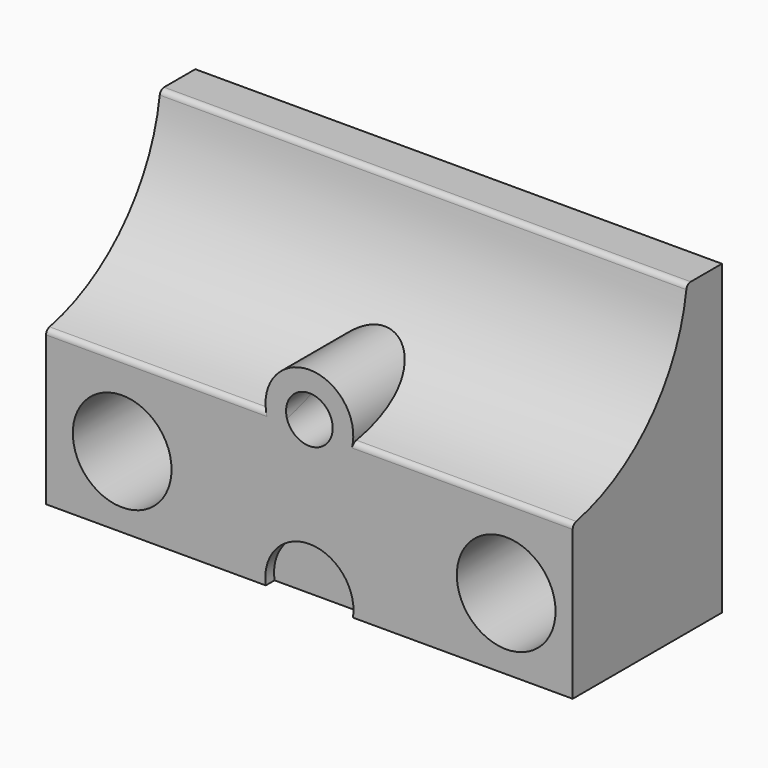
from build123d import *

# Parameters (mm, degrees)
F1_DEPTH      = 152.4
F2_R          = 14.2875
F3_DEPTH      = 101.6
F4_R          = 12.7
F4_R_2        = 6.746875
F5_DEPTH      = 19.05
F6_DEPTH      = 76.2
F7_DEPTH      = 34.925
F8_R          = 12.7653078778
F9_DEPTH      = 3.175
F10_T1_DEPTH  = 159.4216090421
F10_T6_DEPTH  = 70.1643898363
F10_S7_R      = 12.7
F10_T8_DEPTH  = 37
F10_T12_DEPTH = 70.1643898363
F10_S13_R     = 12.7
F10_T14_DEPTH = 37
F11_R         = 3.96875
F12_DEPTH     = 12.7


# Not quite as in the source:
# - a fillet or chamfer that OpenCascade refuses, or shapes differently, is made with other operations: its cross-section is extruded or revolved along the edge and cut away or added
# - a length typed as a fraction of an inch, garbled in the dataset ("3 / 203.2 mm" for 3/8 in), is restored


with BuildPart() as f1:
    # F0 (on Right) → F1 (new body)
    with BuildSketch(Plane.YZ):
        with BuildLine():
            Line((-53.975, 44.45), (-53.975, 0))
            Line((-53.975, 0), (0, 0))
            Line((0, 0), (0, 88.9))
            Line((0, 88.9), (-12.7, 88.9))
            ThreePointArc((-12.7, 88.9), (-25.9749076509, 59.8383071044), (-53.975, 44.45))
        make_face()
    extrude(amount=-F1_DEPTH)

    # F2 (on face) → F3 (cut)
    with BuildSketch(Plane.XZ.offset(53.975)):
        with Locations((-130.3763389587, 20.6375)):
            Circle(F2_R)
        with Locations((-19.2513389587, 20.6375)):
            Circle(F2_R)
    extrude(amount=-F3_DEPTH, mode=Mode.SUBTRACT)

    # F4 (on face) → F5 (cut)
    with BuildSketch(Plane(origin=(0, 0, 0), x_dir=(-1, 0, 0), z_dir=(0, 1, 0))):
        with Locations((76.2, 46.355)):
            Circle(F4_R)
        with Locations((76.2, 46.355)):
            Circle(F4_R_2, mode=Mode.SUBTRACT)
    extrude(amount=-F5_DEPTH, mode=Mode.SUBTRACT)

    # F6 (cut): a face of the model
    f6_faces = [f1.faces().sort_by_distance(p)[0] for p in [
        (-76.2, 0, 46.355),
    ]]
    extrude(f6_faces, amount=-F6_DEPTH, mode=Mode.SUBTRACT)

    # F7 (add, through all): a face of the model
    f7_faces = [f1.faces().sort_by_distance(p)[0] for p in [
        (-63.8592102448, -19.05, 46.355),
    ]]
    extrude(f7_faces, amount=-F7_DEPTH)

    # F8 (on face) → F9 (cut)
    with BuildSketch(Plane.XZ.offset(53.975)):
        with Locations((-76.2, 1.905)):
            Circle(F8_R)
    extrude(amount=-F9_DEPTH, mode=Mode.SUBTRACT)

    # F10: fillet of radius 1.5875 on 3 edges, made by hand

    # F10_s2 → F10_t1 (cut)
    with BuildSketch(Plane.YZ.offset(-155.9108045211)):
        with BuildLine():
            ThreePointArc((-12.8685611865, 87.5274309986), (-12.3394581707, 88.5086101977), (-11.2956781916, 88.9))
            Line((-11.2956781916, 88.9), (-12.7, 88.9))
            ThreePointArc((-12.7, 88.9), (-12.7796098579, 88.2131418999), (-12.8685611865, 87.5274309986))
        make_face()
    extrude(amount=F10_T1_DEPTH, mode=Mode.SUBTRACT)


with BuildPart() as f10_tool4:
    # F10_s5 → F10_t6 (new body)
    with BuildSketch(Plane.YZ.offset(-85.4959611607)):
        with BuildLine():
            ThreePointArc((-52.7151762735, 44.6991736422), (-53.6204522161, 44.1458521426), (-53.975, 43.1458596012))
            Line((-53.975, 43.1458596012), (-53.975, 44.45))
            ThreePointArc((-53.975, 44.45), (-53.3443007137, 44.5706056045), (-52.7151762735, 44.6991736422))
        make_face()
    extrude(amount=-F10_T6_DEPTH)

    # F10_s7 → F10_t8 (cut, symmetric)
    with BuildSketch(Plane.XZ.offset(53.3)):
        with Locations((-76.2, 46.355)):
            Circle(F10_S7_R)
    extrude(amount=F10_T8_DEPTH, both=True, mode=Mode.SUBTRACT)


with BuildPart() as f1_1:
    add(f1.part)

    # F10_t3: cut F10_tool4
    add(f10_tool4.part, mode=Mode.SUBTRACT)


with BuildPart() as f10_tool10:
    # F10_s11 → F10_t12 (new body)
    with BuildSketch(Plane.YZ.offset(3.2603509969)):
        with BuildLine():
            ThreePointArc((-52.7151762735, 44.6991736422), (-53.6204522161, 44.1458521426), (-53.975, 43.1458596012))
            Line((-53.975, 43.1458596012), (-53.975, 44.45))
            ThreePointArc((-53.975, 44.45), (-53.3443007137, 44.5706056045), (-52.7151762735, 44.6991736422))
        make_face()
    extrude(amount=-F10_T12_DEPTH)

    # F10_s13 → F10_t14 (cut, symmetric)
    with BuildSketch(Plane.XZ.offset(53.3)):
        with Locations((-76.2, 46.355)):
            Circle(F10_S13_R)
    extrude(amount=F10_T14_DEPTH, both=True, mode=Mode.SUBTRACT)


with BuildPart() as f1_2:
    add(f1_1.part)

    # F10_t9: cut F10_tool10
    add(f10_tool10.part, mode=Mode.SUBTRACT)

    # F11 (on face) → F12 (cut)
    with BuildSketch(Plane(origin=(0, 0, 0), x_dir=(-1, 0, 0), z_dir=(0, 1, 0))):
        with Locations((20.6375, 60.325)):
            Circle(F11_R)
        with Locations((131.7625, 60.325)):
            Circle(F11_R)
    extrude(amount=-F12_DEPTH, mode=Mode.SUBTRACT)


solid = f1_2.part
